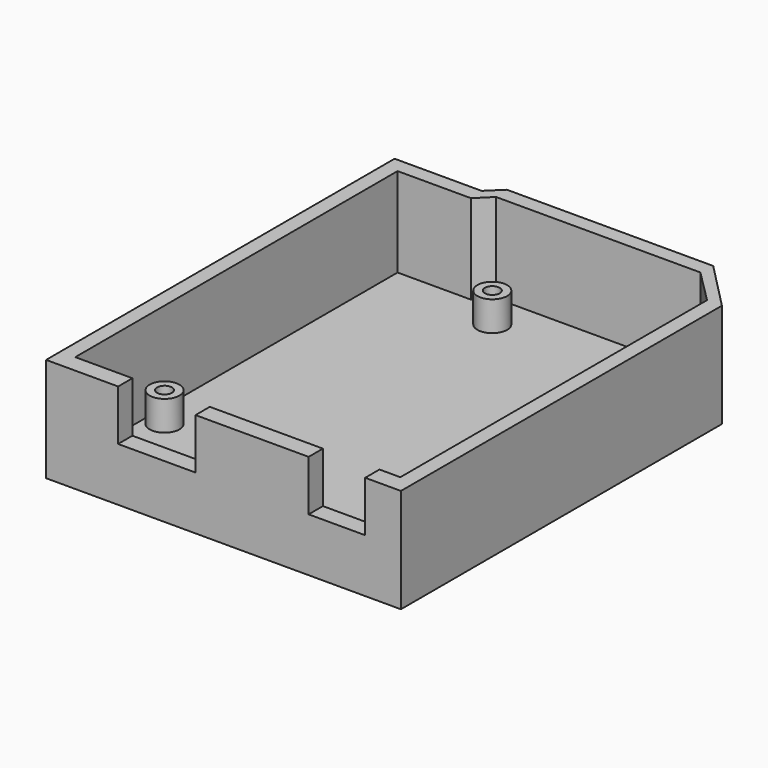
from build123d import *

# Parameters (mm, degrees)
F0_R     = 2.5
F0_W     = 19
F0_H     = 3
F0_W_2   = 13
F0_W_3   = 9.5
F0_R_2   = 1.25
F1_DEPTH = 2.5
F2_DEPTH = 15
F3_DEPTH = 6.5
F4_DEPTH = 2.5
F5_DEPTH = 5


# Not quite as in the source:
# - a feature names something its author has since deleted; it is built from what else it names


with BuildPart() as f1:
    # F0 (on Top) → F1 (new body)
    with BuildSketch(Plane.XY):
        Polygon((27.0149873525, -30.0875452161), (27.0149873525, 34.3124547839), (21.4149873525, 39.9124547839), (-12.9189450768, 39.9124547839), (-15.2438546447, 37.5875452161), (-27.5850126475, 37.5875452161), (-27.5850126475, -30.0875452161), (-17.9850126475, -30.0875452161), (-4.9850126475, -30.0875452161), (14.0149873525, -30.0875452161), (23.5149873525, -30.0875452161), align=None)
        with Locations((-24.5850126475, -15.0875452161)):
            Circle(F0_R, mode=Mode.SUBTRACT)
        with Locations((24.0149873525, -16.0875452161)):
            Circle(F0_R, mode=Mode.SUBTRACT)
        with Locations((-8.6850126475, 33.8492766023)):
            Circle(F0_R, mode=Mode.SUBTRACT)
        with Locations((19.3149873525, 33.8492766023)):
            Circle(F0_R, mode=Mode.SUBTRACT)
        Polygon((21.4149873525, 39.9124547839), (27.0149873525, 34.3124547839), (27.0149873525, -30.0875452161), (29.5149873525, -30.0875452161), (29.5149873525, 34.3124547839), (21.5734839439, 42.4124547839), (-13.0739709929, 42.4124547839), (-15.4701419023, 40.0875452161), (-30.0850126475, 40.0875452161), (-30.0850126475, 10), (-30.0850126475, 5), (-30.0850126475, 0), (-30.0850126475, -5), (-30.0850126475, -30.0875452161), (-27.5850126475, -30.0875452161), (-27.5850126475, 37.5875452161), (-15.2438546447, 37.5875452161), (-12.9189450768, 39.9124547839), align=None)
        with Locations((4.5149873525, -31.5875452161)):
            Rectangle(F0_W, F0_H)
        with Locations((-11.4850126475, -31.5875452161)):
            Rectangle(F0_W_2, F0_H)
        Polygon((-17.9850126475, -33.0875452161), (-17.9850126475, -30.0875452161), (-27.5850126475, -30.0875452161), (-30.0850126475, -30.0875452161), (-30.0850126475, -33.0875452161), align=None)
        with Locations((18.7649873525, -31.5875452161)):
            Rectangle(F0_W_3, F0_H)
        with Locations((19.3149873525, 33.8492766023)):
            Circle(F0_R)
        with Locations((19.3149873525, 33.8492766023)):
            Circle(F0_R_2, mode=Mode.SUBTRACT)
        with Locations((-24.5850126475, -15.0875452161)):
            Circle(F0_R)
        with Locations((-24.5850126475, -15.0875452161)):
            Circle(F0_R_2, mode=Mode.SUBTRACT)
        with Locations((24.0149873525, -16.0875452161)):
            Circle(F0_R)
        with Locations((24.0149873525, -16.0875452161)):
            Circle(F0_R_2, mode=Mode.SUBTRACT)
        with Locations((-8.6850126475, 33.8492766023)):
            Circle(F0_R)
        with Locations((-8.6850126475, 33.8492766023)):
            Circle(F0_R_2, mode=Mode.SUBTRACT)
        Polygon((29.5149873525, -30.0875452161), (27.0149873525, -30.0875452161), (23.5149873525, -30.0875452161), (23.5149873525, -33.0875452161), (29.5149873525, -33.0875452161), align=None)
        with Locations((-24.5850126475, -15.0875452161)):
            Circle(F0_R_2)
        with Locations((24.0149873525, -16.0875452161)):
            Circle(F0_R_2)
        with Locations((-8.6850126475, 33.8492766023)):
            Circle(F0_R_2)
        with Locations((19.3149873525, 33.8492766023)):
            Circle(F0_R_2)
    extrude(amount=-F1_DEPTH)

    # F0 (on Top) → F2 (join)
    with BuildSketch(Plane.XY):
        Polygon((21.4149873525, 39.9124547839), (27.0149873525, 34.3124547839), (27.0149873525, -30.0875452161), (29.5149873525, -30.0875452161), (29.5149873525, 34.3124547839), (21.5734839439, 42.4124547839), (-13.0739709929, 42.4124547839), (-15.4701419023, 40.0875452161), (-30.0850126475, 40.0875452161), (-30.0850126475, 10), (-30.0850126475, 5), (-30.0850126475, 0), (-30.0850126475, -5), (-30.0850126475, -30.0875452161), (-27.5850126475, -30.0875452161), (-27.5850126475, 37.5875452161), (-15.2438546447, 37.5875452161), (-12.9189450768, 39.9124547839), align=None)
        Polygon((-17.9850126475, -33.0875452161), (-17.9850126475, -30.0875452161), (-27.5850126475, -30.0875452161), (-30.0850126475, -30.0875452161), (-30.0850126475, -33.0875452161), align=None)
        with Locations((4.5149873525, -31.5875452161)):
            Rectangle(F0_W, F0_H)
        Polygon((29.5149873525, -30.0875452161), (27.0149873525, -30.0875452161), (23.5149873525, -30.0875452161), (23.5149873525, -33.0875452161), (29.5149873525, -33.0875452161), align=None)
    extrude(amount=F2_DEPTH)

    # F0 (on Top) → F3 (join)
    with BuildSketch(Plane.XY):
        with Locations((-11.4850126475, -31.5875452161)):
            Rectangle(F0_W_2, F0_H)
        with Locations((18.7649873525, -31.5875452161)):
            Rectangle(F0_W_3, F0_H)
    extrude(amount=F3_DEPTH)

    # F0 (on Top) → F4 (join)
    with BuildSketch(Plane.XY):
        with BuildLine():
            Line((-35.0850126475, -5), (-30.0850126475, -5))
            Line((-30.0850126475, -5), (-30.0850126475, 0))
            Line((-30.0850126475, 0), (-30.0850126475, 5))
            Line((-30.0850126475, 5), (-35.0850126475, 5))
            ThreePointArc((-35.0850126475, 5), (-38.6205465534, 3.5355339059), (-40.0850126475, 0))
            ThreePointArc((-40.0850126475, 0), (-38.6205465534, -3.5355339059), (-35.0850126475, -5))
        make_face()
        with Locations((-35.0850126475, 0)):
            Circle(F0_R, mode=Mode.SUBTRACT)
    extrude(amount=-F4_DEPTH)

    # F0 (on Top) → F5 (join)
    with BuildSketch(Plane.XY):
        with Locations((-24.5850126475, -15.0875452161)):
            Circle(F0_R)
        with Locations((-24.5850126475, -15.0875452161)):
            Circle(F0_R_2, mode=Mode.SUBTRACT)
        with Locations((-8.6850126475, 33.8492766023)):
            Circle(F0_R)
        with Locations((-8.6850126475, 33.8492766023)):
            Circle(F0_R_2, mode=Mode.SUBTRACT)
        with Locations((19.3149873525, 33.8492766023)):
            Circle(F0_R)
        with Locations((19.3149873525, 33.8492766023)):
            Circle(F0_R_2, mode=Mode.SUBTRACT)
        with Locations((24.0149873525, -16.0875452161)):
            Circle(F0_R)
        with Locations((24.0149873525, -16.0875452161)):
            Circle(F0_R_2, mode=Mode.SUBTRACT)
    extrude(amount=F5_DEPTH)


solid = f1.part
